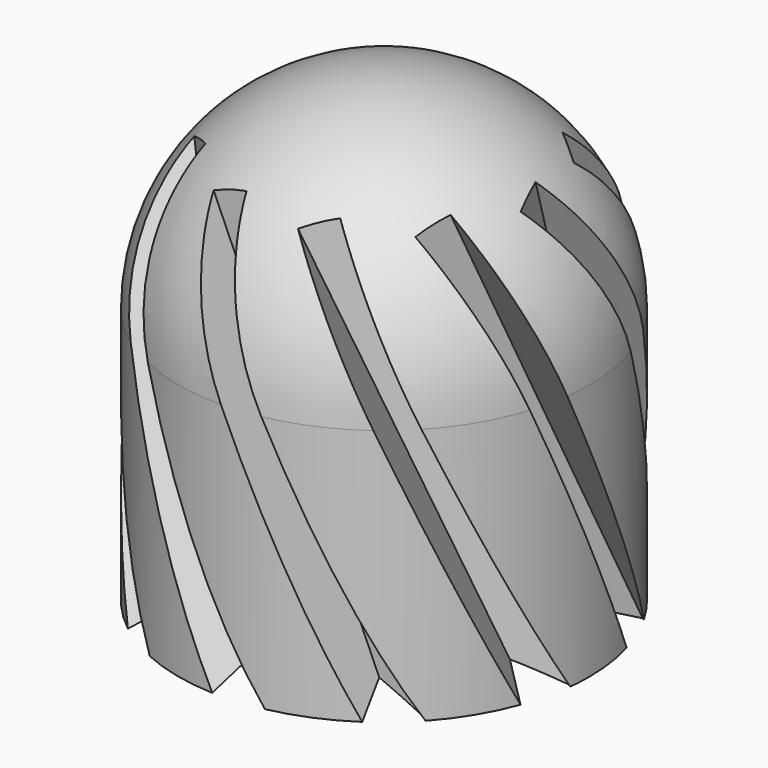
from build123d import *

# Parameters (mm, degrees)
F1_FACE_R       = 7.62
F5_DEPTH        = 25.4
F5_COPIES_COUNT = 10


# Not quite as in the source:
# - a pattern or mirror of a feature is missing from the dataset's text; its kind, count and spacing are read off the source's solid


with BuildPart() as f1:
    # F0 (on Front) → F1 (revolve)
    with BuildSketch(Plane.XZ):
        with BuildLine():
            Line((-7.62, 4.3819724477), (-7.62, -5.1430275523))
            Line((-7.62, -5.1430275523), (0, -5.1430275523))
            Line((0, -5.1430275523), (0, 12.0019724477))
            ThreePointArc((0, 12.0019724477), (-5.3881536726, 9.7701261203), (-7.62, 4.3819724477))
        make_face()
    revolve(axis=Axis((0, 0, 3.4294724477), (0, 0, -1)))

    # F1_face (on face) → F2 section 0
    with BuildSketch(Plane(origin=(0, 0, -5.1430275523), x_dir=(1, 0, 0), z_dir=(0, 0, -1)), mode=Mode.PRIVATE) as f2_s0:
        Circle(F1_FACE_R)
    loft([f2_s0.sketch, Vertex(0, 0, 0)], mode=Mode.SUBTRACT)

    # F4 (on offset) → F5 (cut)
    with BuildSketch(Plane.XZ.offset(5.08)):
        Polygon((6.7222419615, -10.7367794649), (7.8839848078, -10.2236970553), (-11.1258903258, 32.8192645344), (-12.2876331722, 32.3061821249), align=None)
    f5 = extrude(amount=F5_DEPTH, mode=Mode.SUBTRACT)

    # F5_copies: F5 ×10 about axis
    f5_copies_axis = Axis((0, 0, 0), (0, 0, 1))
    for i in range(1, F5_COPIES_COUNT):
        add(f5.rotate(f5_copies_axis, i * 360 / F5_COPIES_COUNT), mode=Mode.SUBTRACT)


solid = f1.part
